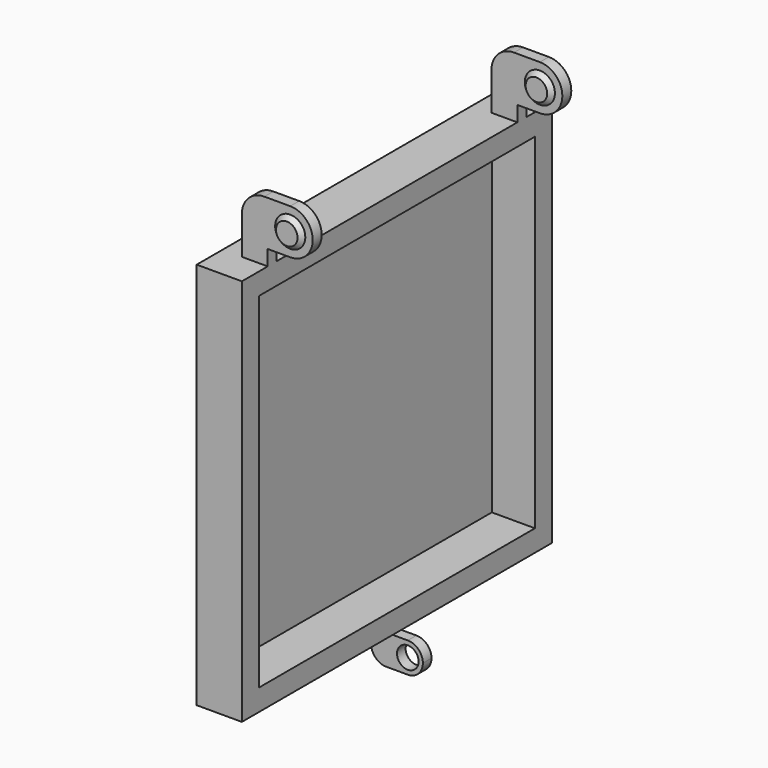
from build123d import *

# Parameters (mm, degrees)
F0_W      = 114.3
F0_H      = 114.3
F0_W_2    = 101.6
F0_H_2    = 101.6
F1_DEPTH  = 12.7
F2_W      = 114.3
F2_H      = 114.3
F3_DEPTH  = 0.6096
F4_W      = 20.8788
F4_H      = 3.302
F5_DEPTH  = 17.78
F6_R      = 6.6294
F8_DEPTH  = 6.35
F9_R      = 6.6294
F10_R     = 4.445
F11_DEPTH = 1.27
F12_R     = 4.445
F13_DEPTH = 1.27
F14_SIZE  = 1.26999
F15_W     = 15.24
F15_H     = 8.89
F16_DEPTH = 1.5875
F17_R     = 4.44499
F18_R     = 3.175
F19_DEPTH = 25.4


# Not quite as in the source:
# - a fillet or chamfer is up to 0.001 mm smaller than in the source, because OpenCascade refuses the exact size
# - a pattern or mirror of a feature is missing from the dataset's text; its kind, count and spacing are read off the source's solid


with BuildPart() as f1:
    # F0 (on Right) → F1 (new body)
    with BuildSketch(Plane.YZ):
        Rectangle(F0_W, F0_H)
        Rectangle(F0_W_2, F0_H_2, mode=Mode.SUBTRACT)
    extrude(amount=F1_DEPTH)

    # F2 (on Right) → F3 (join)
    with BuildSketch(Plane.YZ):
        Rectangle(F2_W, F2_H)
    extrude(amount=-F3_DEPTH)

    # F4 (on face) → F5 (join)
    with BuildSketch(Plane.XY.offset(57.15)):
        with Locations((15.5194, -45.974)):
            Rectangle(F4_W, F4_H)
    f5 = extrude(amount=F5_DEPTH)

    # F5_copies: F5 across plane
    add(f5.mirror(Plane.ZX))

    # F6
    f6_edges = [f1.edges().sort_by_distance(p)[0] for p in [
        (25.9588, -45.974, 74.93),
    ]]
    fillet(f6_edges, radius=F6_R)

    # F7 (on face) → F8 (cut)
    with BuildSketch(Plane.XZ.offset(47.625)):
        with BuildLine():
            ThreePointArc((19.3294, 74.93), (25.9588, 68.3006), (19.3294, 61.6712))
            Line((19.3294, 61.6712), (12.7, 61.6712))
            Line((12.7, 61.6712), (12.7, 57.15))
            Line((12.7, 57.15), (28.7029210806, 51.0326394975))
            Line((28.7029210806, 51.0326394975), (31.0219925225, 81.4440133214))
            Line((31.0219925225, 81.4440133214), (19.3294, 74.93))
        make_face()
    f8 = extrude(amount=-F8_DEPTH, mode=Mode.SUBTRACT)

    # F8_copies: F8 across plane
    add(f8.mirror(Plane.ZX), mode=Mode.SUBTRACT)

    # F9
    f9_edges = [f1.edges().sort_by_distance(p)[0] for p in [
        (5.08, -45.974, 74.93),
        (5.08, 45.974, 74.93),
    ]]
    fillet(f9_edges, radius=F9_R)

    # F10 (on face) → F11 (join)
    with BuildSketch(Plane.XZ.offset(47.625)):
        with Locations((19.3294, 68.3006)):
            Circle(F10_R)
    f11 = extrude(amount=F11_DEPTH)

    # F11_copies: F11 across plane
    add(f11.mirror(Plane.ZX))

    # F12 (on face) → F13 (join)
    with BuildSketch(Plane(origin=(0, -44.323, 0), x_dir=(-1, 0, 0), z_dir=(0, 1, 0))):
        with Locations((-19.3294, 68.3006)):
            Circle(F12_R)
    f13 = extrude(amount=F13_DEPTH)

    # F13_copies: F13 across plane
    add(f13.mirror(Plane.ZX))

    # F14 (size 1.27 in the source; OpenCascade refuses exactly that, so slightly less here)
    f14_edges = [f1.edges().sort_by_distance(p)[0] for p in [
        (14.8844, -48.895, 68.3006),
        (23.7744, -43.053, 68.3006),
        (14.8844, 48.895, 68.3006),
        (23.7744, 43.053, 68.3006),
    ]]
    chamfer(f14_edges, length=F14_SIZE)

    # F15 (on Front) → F16 (join, symmetric)
    with BuildSketch(Plane.XZ):
        with Locations((13.97, -61.595)):
            Rectangle(F15_W, F15_H)
    extrude(amount=F16_DEPTH, both=True)

    # F17 (radius 4.445 in the source; OpenCascade refuses exactly that, so slightly less here)
    f17_edges = [f1.edges().sort_by_distance(p)[0] for p in [
        (21.59, 0, -57.15),
        (21.59, 0, -66.04),
        (6.35, 0, -66.04),
    ]]
    fillet(f17_edges, radius=F17_R)

    # F18 (on face) → F19 (cut)
    with BuildSketch(Plane(origin=(0, 1.5875, 0), x_dir=(-1, 0, 0), z_dir=(0, 1, 0))):
        with Locations((-17.145, -61.595)):
            Circle(F18_R)
    extrude(amount=-F19_DEPTH, mode=Mode.SUBTRACT)


solid = f1.part
